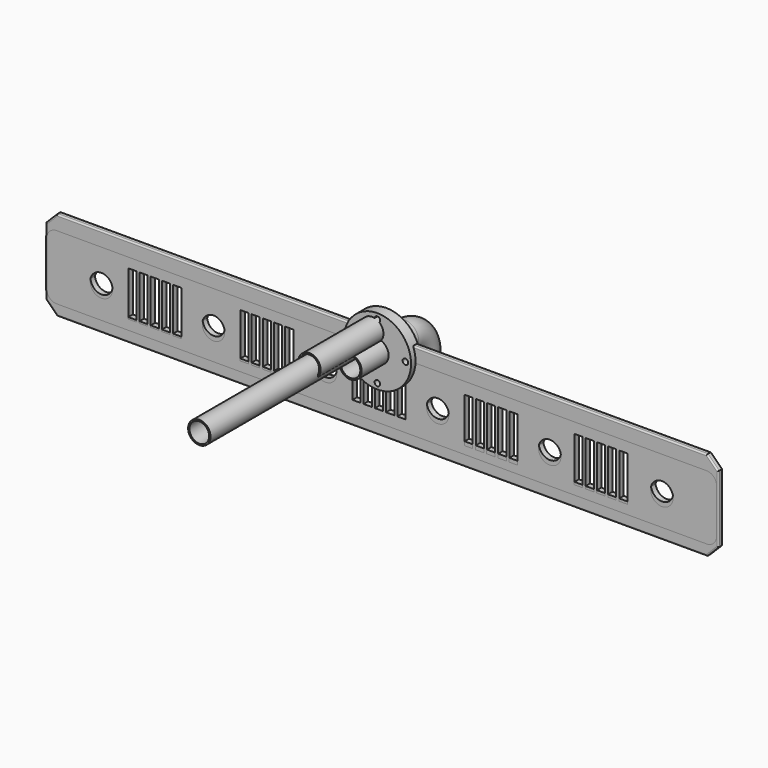
from build123d import *

# Parameters (mm, degrees)
F0_R           = 38.1
F0_R_2         = 9.525
F1_DEPTH       = 12.7
F2_R           = 12.7
F2_R_2         = 9.525
F3_DEPTH       = 6.35
F5_D           = 3.175
F5_CBORE_D     = 6.35
F5_CBORE_DEPTH = 6.35
F6_R           = 23.8125
F6_R_2         = 22.225
F7_DEPTH       = 1.905
F8_R           = 12.7
F8_R_2         = 11.1125
F9_DEPTH       = 50.8
F10_R          = 12.7
F10_R_2        = 11.1125
F11_DEPTH      = 101.6
F12_R          = 12.7
F12_R_2        = 11.1125
F13_DEPTH      = 254
F14_R          = 15.875
F14_R_2        = 11.1125
F17_R          = 12.7
F18_DEPTH      = 12.7
F19_R          = 12.7
F20_DEPTH      = 12.7
F21_W          = 762
F21_H          = 101.6
F21_R          = 12.7
F22_DEPTH      = 6.35
F23_W          = 9.525
F23_H          = 50.8
F24_DEPTH      = 73.1173910971
F25_SIZE       = 12.7
F26_R          = 1.6002
F27_W          = 762
F27_H          = 76.2
F27_R          = 12.7
F28_DEPTH      = 6.35
F29_W          = 9.525
F29_H          = 50.8
F30_DEPTH      = 73.1173910971
F31_R          = 12.7
F32_R          = 1.6002


with BuildPart() as f1:
    # F0 (on Front) → F1 (new body)
    with BuildSketch(Plane.XZ):
        Circle(F0_R)
        Circle(F0_R_2, mode=Mode.SUBTRACT)
    extrude(amount=F1_DEPTH)

    # F2 (on face) → F3 (cut)
    with BuildSketch(Plane.XZ.offset(12.7)):
        Circle(F2_R)
        Circle(F2_R_2, mode=Mode.SUBTRACT)
    extrude(amount=-F3_DEPTH, mode=Mode.SUBTRACT)

    # F5 (through all)
    with Locations(Plane.XZ.offset(12.7)):
        with Locations((0, 31.75), (-31.75, 0), (31.75, 0), (0, -31.75)):
            CounterBoreHole(F5_D / 2, F5_CBORE_D / 2, F5_CBORE_DEPTH)

    # F6 (on face) → F7 (cut)
    with BuildSketch(Plane(origin=(0, 0, 0), x_dir=(-1, 0, 0), z_dir=(0, 1, 0))):
        Circle(F6_R)
        Circle(F6_R_2, mode=Mode.SUBTRACT)
    extrude(amount=-F7_DEPTH, mode=Mode.SUBTRACT)


with BuildPart() as f9:
    # F8 (on Front) → F9 (new body)
    with BuildSketch(Plane.XZ):
        Circle(F8_R)
        Circle(F8_R_2, mode=Mode.SUBTRACT)
    extrude(amount=F9_DEPTH)


with BuildPart() as f11:
    # F10 (on Front) → F11 (new body)
    with BuildSketch(Plane.XZ):
        with Locations((-5.8710384183, 19.78828758)):
            Circle(F10_R)
        with Locations((-5.8710384183, 19.78828758)):
            Circle(F10_R_2, mode=Mode.SUBTRACT)
    extrude(amount=F11_DEPTH)


with BuildPart() as f13:
    # F12 (on Front) → F13 (new body)
    with BuildSketch(Plane.XZ):
        with Locations((-8.7111480534, 14.297645539)):
            Circle(F12_R)
        with Locations((-8.7111480534, 14.297645539)):
            Circle(F12_R_2, mode=Mode.SUBTRACT)
    extrude(amount=F13_DEPTH)


with BuildPart() as f16:
    # F16: sweep along a path in F15
    with BuildLine(Plane.YZ) as f16_path:
        Line((50.8, -50.8), (50.8, -25.4))
        ThreePointArc((50.8, -25.4), (43.3605122421, -7.4394877579), (25.4, 0))
        Line((25.4, 0), (0, 0))
    # F14 (on Front) → F16 (sweep)
    with BuildSketch(Plane.XZ):
        with Locations((0.3774386423, 0.0913909971)):
            Circle(F14_R)
        with Locations((0.3774386423, 0.0913909971)):
            Circle(F14_R_2, mode=Mode.SUBTRACT)
    sweep(path=f16_path.line)

    # F17 (on Front) → F18 (cut)
    with BuildSketch(Plane.XZ):
        Circle(F17_R)
    extrude(amount=-F18_DEPTH, mode=Mode.SUBTRACT)

    # F19 (on face) → F20 (cut)
    with BuildSketch(Plane(origin=(0, 0, -50.8), x_dir=(1, 0, 0), z_dir=(0, 0, -1))):
        with Locations((0.3774386423, -50.8913909971)):
            Circle(F19_R)
    extrude(amount=-F20_DEPTH, mode=Mode.SUBTRACT)


with BuildPart() as f22:
    # F21 (on Front) → F22 (new body)
    with BuildSketch(Plane.XZ):
        with Locations((0, -36.4666409148)):
            Rectangle(F21_W, F21_H)
        with Locations((-317.5, -36.4666409148)):
            Circle(F21_R, mode=Mode.SUBTRACT)
        with Locations((-63.5, -36.4666409148)):
            Circle(F21_R, mode=Mode.SUBTRACT)
        with Locations((-190.5, -36.4666409148)):
            Circle(F21_R, mode=Mode.SUBTRACT)
        with Locations((63.5, -36.4666409148)):
            Circle(F21_R, mode=Mode.SUBTRACT)
        with Locations((190.5, -36.4666409148)):
            Circle(F21_R, mode=Mode.SUBTRACT)
        with Locations((317.5, -36.4666409148)):
            Circle(F21_R, mode=Mode.SUBTRACT)
    extrude(amount=F22_DEPTH)

    # F23 (on face) → F24 (cut, through all)
    with BuildSketch(Plane.XZ.offset(6.35)):
        with Locations((-282.5623, -36.4666409148)):
            Rectangle(F23_W, F23_H)
        with Locations((-269.8623, -36.4666409148)):
            Rectangle(F23_W, F23_H)
        with Locations((-257.1623, -36.4666409148)):
            Rectangle(F23_W, F23_H)
        with Locations((-244.4623, -36.4666409148)):
            Rectangle(F23_W, F23_H)
        with Locations((-231.7623, -36.4666409148)):
            Rectangle(F23_W, F23_H)
        with Locations((-155.5623, -36.4666409148)):
            Rectangle(F23_W, F23_H)
        with Locations((-142.8623, -36.4666409148)):
            Rectangle(F23_W, F23_H)
        with Locations((-130.1623, -36.4666409148)):
            Rectangle(F23_W, F23_H)
        with Locations((-117.4623, -36.4666409148)):
            Rectangle(F23_W, F23_H)
        with Locations((-104.7623, -36.4666409148)):
            Rectangle(F23_W, F23_H)
        with Locations((-28.5623, -36.4666409148)):
            Rectangle(F23_W, F23_H)
        with Locations((-15.8623, -36.4666409148)):
            Rectangle(F23_W, F23_H)
        with Locations((-3.1623, -36.4666409148)):
            Rectangle(F23_W, F23_H)
        with Locations((9.5377, -36.4666409148)):
            Rectangle(F23_W, F23_H)
        with Locations((22.2377, -36.4666409148)):
            Rectangle(F23_W, F23_H)
        with Locations((98.4377, -36.4666409148)):
            Rectangle(F23_W, F23_H)
        with Locations((111.1377, -36.4666409148)):
            Rectangle(F23_W, F23_H)
        with Locations((123.8377, -36.4666409148)):
            Rectangle(F23_W, F23_H)
        with Locations((136.5377, -36.4666409148)):
            Rectangle(F23_W, F23_H)
        with Locations((149.2377, -36.4666409148)):
            Rectangle(F23_W, F23_H)
        with Locations((222.8977, -36.4666409148)):
            Rectangle(F23_W, F23_H)
        with Locations((235.5977, -36.4666409148)):
            Rectangle(F23_W, F23_H)
        with Locations((248.2977, -36.4666409148)):
            Rectangle(F23_W, F23_H)
        with Locations((260.9977, -36.4666409148)):
            Rectangle(F23_W, F23_H)
        with Locations((273.6977, -36.4666409148)):
            Rectangle(F23_W, F23_H)
    extrude(amount=-F24_DEPTH, mode=Mode.SUBTRACT)

    # F25
    f25_edges = [f22.edges().sort_by_distance(p)[0] for p in [
        (-381, -3.175, 14.333359),
        (-381, -3.175, -87.266641),
        (381, -3.175, 14.333359),
        (381, -3.175, -87.266641),
    ]]
    chamfer(f25_edges, length=F25_SIZE)

    # F26
    f26_edges = [f22.edges().sort_by_distance(p)[0] for p in [
        (-374.65, -6.35, 7.983359),
        (-374.65, -6.35, -80.916641),
        (374.65, -6.35, 7.983359),
        (374.65, -6.35, -80.916641),
        (0, -6.35, 14.333359),
        (0, -6.35, -87.266641),
        (-381, -6.35, -36.466641),
        (381, -6.35, -36.466641),
        (0, 0, 14.333359),
        (374.65, 0, 7.983359),
        (381, 0, -36.466641),
        (374.65, 0, -80.916641),
        (0, 0, -87.266641),
        (-374.65, 0, 7.983359),
        (-381, 0, -36.466641),
        (-374.65, 0, -80.916641),
    ]]
    fillet(f26_edges, radius=F26_R)


with BuildPart() as f28:
    # F27 (on Front) → F28 (new body)
    with BuildSketch(Plane.XZ):
        with Locations((-0.2840571105, -38.5347231889)):
            Rectangle(F27_W, F27_H)
        with Locations((-317.7840571105, -40.3055138886)):
            Circle(F27_R, mode=Mode.SUBTRACT)
        with Locations((-190.7840571105, -41.5128655732)):
            Circle(F27_R, mode=Mode.SUBTRACT)
        with Locations((-63.7840571105, -41.5128655732)):
            Circle(F27_R, mode=Mode.SUBTRACT)
        with Locations((63.2159428895, -41.5128655732)):
            Circle(F27_R, mode=Mode.SUBTRACT)
        with Locations((190.2159428895, -41.5128655732)):
            Circle(F27_R, mode=Mode.SUBTRACT)
        with Locations((317.2159428895, -41.5128655732)):
            Circle(F27_R, mode=Mode.SUBTRACT)
    extrude(amount=F28_DEPTH)

    # F29 (on face) → F30 (cut, through all)
    with BuildSketch(Plane.XZ.offset(6.35)):
        with Locations((-282.8463571105, -38.5347231889)):
            Rectangle(F29_W, F29_H)
        with Locations((-270.1463571105, -38.5347231889)):
            Rectangle(F29_W, F29_H)
        with Locations((-257.4463571105, -38.5347231889)):
            Rectangle(F29_W, F29_H)
        with Locations((-244.7463571105, -38.5347231889)):
            Rectangle(F29_W, F29_H)
        with Locations((-232.0463571105, -38.5347231889)):
            Rectangle(F29_W, F29_H)
        with Locations((-155.8463571105, -38.915775997)):
            Rectangle(F29_W, F29_H)
        with Locations((-143.1463571105, -38.915775997)):
            Rectangle(F29_W, F29_H)
        with Locations((-130.4463571105, -38.915775997)):
            Rectangle(F29_W, F29_H)
        with Locations((-117.7463571105, -38.915775997)):
            Rectangle(F29_W, F29_H)
        with Locations((-105.0463571105, -38.915775997)):
            Rectangle(F29_W, F29_H)
        with Locations((-28.8463571105, -36.4282320267)):
            Rectangle(F29_W, F29_H)
        with Locations((-16.1463571105, -36.4282320267)):
            Rectangle(F29_W, F29_H)
        with Locations((-3.4463571105, -36.4282320267)):
            Rectangle(F29_W, F29_H)
        with Locations((9.2536428895, -36.4282320267)):
            Rectangle(F29_W, F29_H)
        with Locations((21.9536428895, -36.4282320267)):
            Rectangle(F29_W, F29_H)
        with Locations((98.1536428895, -40.7814311808)):
            Rectangle(F29_W, F29_H)
        with Locations((110.8536428895, -40.7814311808)):
            Rectangle(F29_W, F29_H)
        with Locations((123.5536428895, -40.7814311808)):
            Rectangle(F29_W, F29_H)
        with Locations((136.2536428895, -40.7814311808)):
            Rectangle(F29_W, F29_H)
        with Locations((148.9536428895, -40.7814311808)):
            Rectangle(F29_W, F29_H)
        with Locations((222.6136428895, -39.3401163643)):
            Rectangle(F29_W, F29_H)
        with Locations((235.3136428895, -39.3401163643)):
            Rectangle(F29_W, F29_H)
        with Locations((248.0136428895, -39.3401163643)):
            Rectangle(F29_W, F29_H)
        with Locations((260.7136428895, -39.3401163643)):
            Rectangle(F29_W, F29_H)
        with Locations((273.4136428895, -39.3401163643)):
            Rectangle(F29_W, F29_H)
    extrude(amount=-F30_DEPTH, mode=Mode.SUBTRACT)

    # F31
    f31_edges = [f28.edges().sort_by_distance(p)[0] for p in [
        (-381.284057, -3.175, -0.434723),
        (-381.284057, -3.175, -76.634723),
        (380.715943, -3.175, -0.434723),
        (380.715943, -3.175, -76.634723),
    ]]
    fillet(f31_edges, radius=F31_R)

    # F32
    f32_edges = [f28.edges().sort_by_distance(p)[0] for p in [
        (-0.284057, -6.35, -0.434723),
        (-0.284057, 0, -0.434723),
        (380.715943, 0, -38.534723),
        (-381.284057, 0, -38.534723),
        (380.715943, -6.35, -38.534723),
        (-381.284057, -6.35, -38.534723),
    ]]
    fillet(f32_edges, radius=F32_R)


solid = Compound([f1.part, f9.part, f11.part, f13.part, f16.part, f22.part, f28.part])
